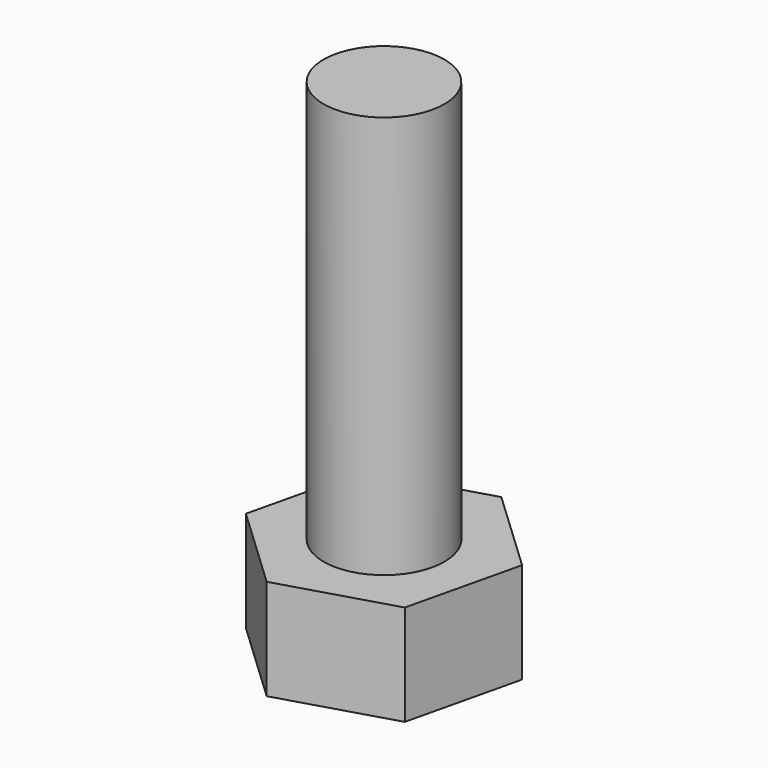
from build123d import *

# Parameters (mm, degrees)
F0_R     = 3
F1_DEPTH = 20
F2_R     = 3
F3_DEPTH = 5


with BuildPart() as f1:
    # F0 (on Top) → F1 (new body)
    with BuildSketch(Plane.XY):
        Circle(F0_R)
    extrude(amount=F1_DEPTH)

    # F2 (on face) → F3 (join)
    with BuildSketch(Plane(origin=(0, 0, 0), x_dir=(1, 0, 0), z_dir=(0, 0, -1))):
        Polygon((1.3301522364, -5.6181872843), (5.5305690296, -1.6571480145), (4.2004167932, 3.9610392698), (-1.3301522364, 5.6181872843), (-5.5305690296, 1.6571480145), (-4.2004167932, -3.9610392698), align=None)
        Circle(F2_R, mode=Mode.SUBTRACT)
        Circle(F2_R)
    extrude(amount=F3_DEPTH)


solid = f1.part
